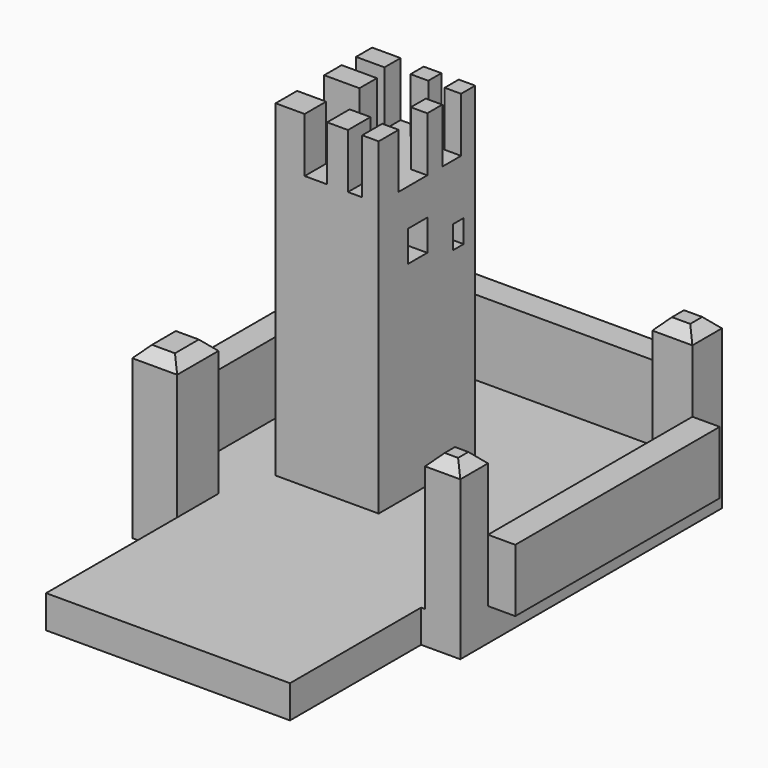
from build123d import *

# Parameters (mm, degrees)
F0_W      = 152.5124907494
F0_H      = 152.087032795
F1_DEPTH  = 2.54
F2_W      = 20.8487436175
F2_H      = 24.0208171308
F3_DEPTH  = 76.2
F2_W_2    = 17.8325101733
F2_H_2    = 23.2902280986
F4_DEPTH  = 76.2
F2_W_3    = 16.3801498711
F2_H_3    = 16.0977393389
F2_W_4    = 18.6377316713
F2_H_4    = 17.1602889895
F5_DEPTH  = 76.2
F6_DEPTH  = 12.7
F6_FACE_W = 20.8487436175
F6_FACE_H = 24.0208171308
F7_DEPTH  = 12.7
F8_SIZE   = 5.08
F12_W     = 118.8290044665
F12_H     = 29.21
F13_DEPTH = 12.7
F15_W     = 115.0837503374
F15_H     = 34.9880257642
F16_DEPTH = 12.7
F17_W     = 104.7759875655
F17_H     = 33.3026150262
F18_DEPTH = 12.7
F19_W     = 113.4291402996
F19_H     = 15.24
F20_DEPTH = 76.2
F22_W     = 47.9301847517
F22_H     = 56.1127942055
F23_DEPTH = 127
F24_W     = 13.509940356
F24_H     = 12.4862398952
F25_DEPTH = 25.4
F24_W_2   = 16.3891837001
F24_H_2   = 10.1510994136
F26_DEPTH = 25.4
F24_W_3   = 13.2220201194
F24_H_3   = 9.3634463847
F27_DEPTH = 25.4
F24_W_4   = 8.2599930465
F24_H_4   = 7.6358895749
F28_DEPTH = 25.4
F24_W_5   = 7.6431990601
F24_H_5   = 8.2117523998
F29_DEPTH = 25.4
F24_H_6   = 8.7114600465
F30_DEPTH = 25.4
F24_H_7   = 11.6224680096
F31_DEPTH = 25.4
F24_W_6   = 9.6996221691
F24_H_8   = 13.0620943382
F32_DEPTH = 25.4
F33_W     = 11.1384242773
F33_H     = 14.4351422787
F34_DEPTH = 12.7
F33_W_2   = 6.1493515968
F33_H_2   = 10.6694698334
F35_DEPTH = 25.4


# Not quite as in the source:
# - two fillets or chamfers of one size are made in one step
# - the program builds the solid bodies; features that only make, move or delete a surface that nothing else refers to are left out


with BuildPart() as f1:
    # F0 (on Top) → F1 (new body)
    with BuildSketch(Plane.XY):
        with Locations((0.1670345664, -0.2893134952)):
            Rectangle(F0_W, F0_H)
    extrude(amount=F1_DEPTH)

    # F2 (on face) → F3 (join)
    with BuildSketch(Plane.XY.offset(2.54)):
        with Locations((-65.6648389995, -64.3224213272)):
            Rectangle(F2_W, F2_H)
    extrude(amount=F3_DEPTH)

    # F2 (on face) → F4 (join)
    with BuildSketch(Plane.XY.offset(2.54)):
        with Locations((-67.1729557216, 64.109088853)):
            Rectangle(F2_W_2, F2_H_2)
    extrude(amount=F4_DEPTH)

    # F2 (on face) → F5 (join)
    with BuildSketch(Plane.XY.offset(2.54)):
        with Locations((68.2332050055, -68.2839602232)):
            Rectangle(F2_W_3, F2_H_3)
        with Locations((67.1044141054, 67.1740584075)):
            Rectangle(F2_W_4, F2_H_4)
    extrude(amount=F5_DEPTH)

    # F6 (cut): a face of the model
    f6_faces = [f1.faces().sort_by_distance(p)[0] for p in [
        (-65.6648389995, -64.3224213272, 78.74),
    ]]
    extrude(f6_faces, amount=-F6_DEPTH, mode=Mode.SUBTRACT)

    # F2 (on face) + F6_face (on face) → F7 (join)
    with BuildSketch(Plane.XY.offset(2.54)):
        Polygon((-55.2404671907, -52.3120127618), (-55.2404671907, -76.3328298926), (60.04313007, -76.3328298926), (60.04313007, -60.2350905538), (76.4232799411, -60.2350905538), (76.4232799411, 58.5939139128), (57.7855482697, 58.5939139128), (57.7855482697, 75.7542029023), (-58.256700635, 75.7542029023), (-58.256700635, 52.4639748037), (-76.0892108083, 52.4639748037), (-76.0892108083, -52.3120127618), align=None)
    with BuildSketch(Plane(origin=(-65.6648389995, -64.3224213272, 66.04), x_dir=(1, 0, 0), z_dir=(0, 0, 1))):
        Rectangle(F6_FACE_W, F6_FACE_H)
    extrude(amount=F7_DEPTH)

    # F8
    f8_edges = [f1.edges().sort_by_distance(p)[0] for p in [
        (-65.664839, -76.33283, 78.74),
        (-76.089211, -64.322421, 78.74),
        (-76.089211, 64.109089, 78.74),
        (76.42328, -68.28396, 78.74),
        (76.42328, 67.174058, 78.74),
        (67.104414, 58.593914, 78.74),
        (67.104414, 75.754203, 78.74),
        (57.785548, 67.174058, 78.74),
        (68.233205, -60.235091, 78.74),
        (60.04313, -68.28396, 78.74),
        (68.233205, -76.33283, 78.74),
        (-55.240467, -64.322421, 78.74),
        (-65.664839, -52.312013, 78.74),
        (-58.256701, 64.109089, 78.74),
        (-67.172956, 52.463975, 78.74),
        (-67.172956, 75.754203, 78.74),
    ]]
    chamfer(f8_edges, length=F8_SIZE)

    # F19 (on face) → F20 (join)
    with BuildSketch(Plane.XZ.offset(76.3328298926)):
        with Locations((1.474102959, 7.62)):
            Rectangle(F19_W, F19_H)
    extrude(amount=F20_DEPTH)

    # F22 (on face) → F23 (join)
    with BuildSketch(Plane.XY.offset(15.24)):
        with Locations((-23.9650923759, -0.1920359209)):
            Rectangle(F22_W, F22_H)
    extrude(amount=F23_DEPTH)

    # F24 (on face) → F25 (join)
    with BuildSketch(Plane.XY.offset(142.24)):
        with Locations((-41.1752145737, -22.0053130761)):
            Rectangle(F24_W, F24_H)
    extrude(amount=F25_DEPTH)

    # F24 (on face) → F26 (join)
    with BuildSketch(Plane.XY.offset(142.24)):
        with Locations((-39.7355929017, 5.0755497068)):
            Rectangle(F24_W_2, F24_H_2)
    extrude(amount=F26_DEPTH)

    # F24 (on face) → F27 (join)
    with BuildSketch(Plane.XY.offset(142.24)):
        with Locations((-41.319174692, 23.1826379895)):
            Rectangle(F24_W_3, F24_H_3)
    extrude(amount=F27_DEPTH)

    # F24 (on face) → F28 (join)
    with BuildSketch(Plane.XY.offset(142.24)):
        with Locations((-19.8350958526, 24.0464163944)):
            Rectangle(F24_W_4, F24_H_4)
    extrude(amount=F28_DEPTH)

    # F24 (on face) → F29 (join)
    with BuildSketch(Plane.XY.offset(142.24)):
        with Locations((-3.8215995301, 23.758484982)):
            Rectangle(F24_W_5, F24_H_5)
    extrude(amount=F29_DEPTH)

    # F24 (on face) → F30 (join)
    with BuildSketch(Plane.XY.offset(142.24)):
        with Locations((-3.8215995301, 4.3557300232)):
            Rectangle(F24_W_5, F24_H_6)
    extrude(amount=F30_DEPTH)

    # F24 (on face) → F31 (join)
    with BuildSketch(Plane.XY.offset(142.24)):
        with Locations((-3.8215995301, -22.4371990189)):
            Rectangle(F24_W_5, F24_H_7)
    extrude(amount=F31_DEPTH)

    # F24 (on face) → F32 (join)
    with BuildSketch(Plane.XY.offset(142.24)):
        with Locations((-19.1152812913, -21.7173858546)):
            Rectangle(F24_W_6, F24_H_8)
    extrude(amount=F32_DEPTH)

    # F33 (on face) → F34 (cut)
    with BuildSketch(Plane.YZ):
        with Locations((-5.5692121387, 117.7433207631)):
            Rectangle(F33_W, F33_H)
    extrude(amount=-F34_DEPTH, mode=Mode.SUBTRACT)

    # F33 (on face) → F35 (cut)
    with BuildSketch(Plane.YZ):
        with Locations((18.0709660053, 110.8395680785)):
            Rectangle(F33_W_2, F33_H_2)
    extrude(amount=-F35_DEPTH, mode=Mode.SUBTRACT)


with BuildPart() as f13:
    # F12 (on face) → F13 (new body)
    with BuildSketch(Plane.YZ.offset(76.4232799411)):
        with Locations((-0.8205883205, 29.845)):
            Rectangle(F12_W, F12_H)
    extrude(amount=F13_DEPTH)


with BuildPart() as f16:
    # F15 (on face) → F16 (new body)
    with BuildSketch(Plane(origin=(0, 75.7542029023, 0), x_dir=(-1, 0, 0), z_dir=(0, 1, 0))):
        with Locations((-0.2436731011, 32.7340128821)):
            Rectangle(F15_W, F15_H)
    extrude(amount=F16_DEPTH)


with BuildPart() as f18:
    # F17 (on face) → F18 (new body)
    with BuildSketch(Plane(origin=(-76.0892108083, 0, 0), x_dir=(0, -1, 0), z_dir=(-1, 0, 0))):
        with Locations((-0.0759810209, 31.8913075131)):
            Rectangle(F17_W, F17_H)
    extrude(amount=F18_DEPTH)


solid = Compound([f1.part, f13.part, f16.part, f18.part])
